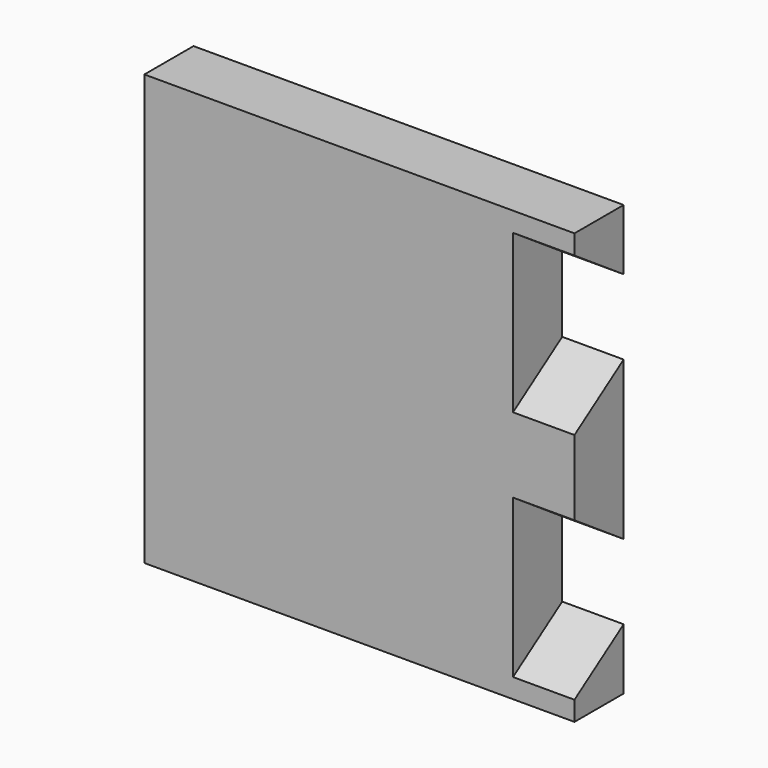
from build123d import *

# Parameters (mm, degrees)
F0_W     = 120
F0_H     = 140
F0_W_2   = 20
F1_DEPTH = 20
F3_DEPTH = 20
F5_DEPTH = 10


# Not quite as in the source:
# - ends of sketch curves that miss each other by under 0.0002 mm in the source are joined


with BuildPart() as f1:
    # F0 (on Front) → F1 (new body)
    with BuildSketch(Plane.XZ):
        with Locations((-60, 70)):
            Rectangle(F0_W, F0_H)
        with Locations((-130, 70)):
            Rectangle(F0_W_2, F0_H)
    extrude(amount=F1_DEPTH)

    # F2 (on face) → F3 (cut)
    with BuildSketch(Plane.YZ):
        Polygon((-20, 133.6477049324), (-20, 82.2157338262), (0, 95.7159893793), (0, 120.1474493793), align=None)
        Polygon((0, 44.2840144469), (-20, 57.78427), (-20, 6.3522950676), (0, 19.8525506207), align=None)
    extrude(amount=-F3_DEPTH, mode=Mode.SUBTRACT)

    # F4 (on face) → F5 (cut)
    with BuildSketch(Plane(origin=(-140, 0, 0), x_dir=(0, -1, 0), z_dir=(-1, 0, 0))):
        with BuildLine():
            ThreePointArc((15, 75.9070515633), (10, 80.9070515633), (5, 75.9070515633))
            Line((5, 75.9070515633), (15, 75.9070515633))
        make_face()
        with BuildLine():
            Line((15, 75.9070515633), (5, 75.9070515633))
            ThreePointArc((5, 75.9070515633), (10, 70.9070515633), (15, 75.9070515633))
        make_face()
        with BuildLine():
            ThreePointArc((15, 33.7962135673), (10, 38.7962135673), (5, 33.7962135673))
            Line((5, 33.7962135673), (15, 33.7962135673))
        make_face()
        with BuildLine():
            Line((15, 33.7962135673), (5, 33.7962135673))
            ThreePointArc((5, 33.7962135673), (10, 28.7962135673), (15, 33.7962135673))
        make_face()
        with BuildLine():
            ThreePointArc((15, 118.0178895593), (10, 123.0178895593), (5, 118.0178895593))
            Line((5, 118.0178895593), (15, 118.0178895593))
        make_face()
        with BuildLine():
            Line((15, 118.0178895593), (5, 118.0178895593))
            ThreePointArc((5, 118.0178895593), (10, 113.0178895593), (15, 118.0178895593))
        make_face()
    extrude(amount=-F5_DEPTH, mode=Mode.SUBTRACT)


solid = f1.part
